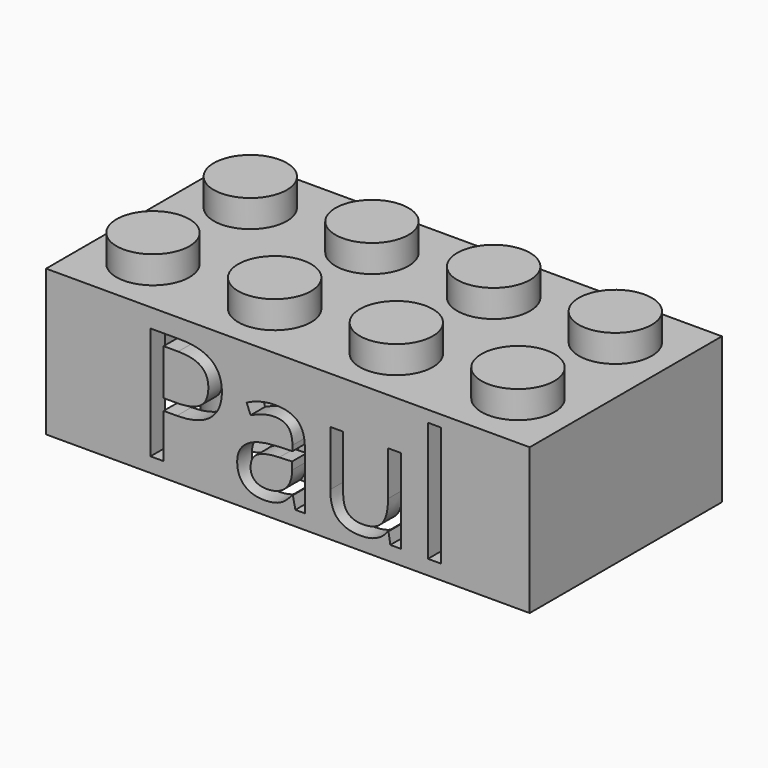
from build123d import *

# Parameters (mm, degrees)
F0_W          = 31.8
F0_H          = 15.8
F1_DEPTH      = 9.6
F2_W          = 29.4
F2_H          = 13.4
F3_DEPTH      = 8.4
F4_R          = 2.4
F5_DEPTH      = 1.8
F6_R          = 1.3
F7_DEPTH      = 1.2
F8_R          = 3.255
F8_R_2        = 2.4
F9_DEPTH      = 8.4
F10_W         = 0.6
F10_H         = 0.3
F11_DEPTH     = 8.4
F12_W         = 0.3
F12_H         = 0.6
F13_DEPTH     = 8.4
F14_W         = 0.6
F14_H         = 4
F15_DEPTH     = 6.4
F16_W         = 0.6
F16_H         = 4
F17_DEPTH     = 6.4
F18_TEXT_SIZE = 10.368521
F19_DEPTH     = 1.2


# Not quite as in the source:
# - Text() gives the source's letters only with a copy of the font that has no kerning and outlines rounded to 1/6400 em; it was checked with that copy


with BuildPart() as f1:
    # F0 (on Top) → F1 (new body)
    with BuildSketch(Plane.XY):
        Rectangle(F0_W, F0_H)
    extrude(amount=F1_DEPTH)

    # F2 (on face) → F3 (cut)
    with BuildSketch(Plane(origin=(0, 0, 0), x_dir=(1, 0, 0), z_dir=(0, 0, -1))):
        Rectangle(F2_W, F2_H)
    extrude(amount=-F3_DEPTH, mode=Mode.SUBTRACT)

    # F4 (on face) → F5 (join)
    with BuildSketch(Plane.XY.offset(9.6)):
        with Locations((-11.95, 3.95)):
            Circle(F4_R)
        with Locations((-11.95, -4.05)):
            Circle(F4_R)
        with Locations((-3.95, 3.95)):
            Circle(F4_R)
        with Locations((-3.95, -4.05)):
            Circle(F4_R)
        with Locations((4.05, 3.95)):
            Circle(F4_R)
        with Locations((4.05, -4.05)):
            Circle(F4_R)
        with Locations((12.05, 3.95)):
            Circle(F4_R)
        with Locations((12.05, -4.05)):
            Circle(F4_R)
    extrude(amount=F5_DEPTH)

    # F6 (on face) → F7 (cut)
    with BuildSketch(Plane(origin=(0, 0, 8.4), x_dir=(1, 0, 0), z_dir=(0, 0, -1))):
        with Locations((-11.95, 3.95)):
            Circle(F6_R)
        with Locations((-11.95, -4.05)):
            Circle(F6_R)
        with Locations((-3.95, 3.95)):
            Circle(F6_R)
        with Locations((-3.95, -4.05)):
            Circle(F6_R)
        with Locations((4.05, 3.95)):
            Circle(F6_R)
        with Locations((4.05, -4.05)):
            Circle(F6_R)
        with Locations((12.05, 3.95)):
            Circle(F6_R)
        with Locations((12.05, -4.05)):
            Circle(F6_R)
    extrude(amount=-F7_DEPTH, mode=Mode.SUBTRACT)

    # F8 (on face) → F9 (join, through all)
    with BuildSketch(Plane(origin=(0, 0, 8.4), x_dir=(1, 0, 0), z_dir=(0, 0, -1))):
        with Locations((-7.95, -0.05)):
            Circle(F8_R)
        with Locations((-7.95, -0.05)):
            Circle(F8_R_2, mode=Mode.SUBTRACT)
        with Locations((0.05, -0.05)):
            Circle(F8_R)
        with Locations((0.05, -0.05)):
            Circle(F8_R_2, mode=Mode.SUBTRACT)
        with Locations((8.05, -0.05)):
            Circle(F8_R)
        with Locations((8.05, -0.05)):
            Circle(F8_R_2, mode=Mode.SUBTRACT)
    extrude(amount=F9_DEPTH)

    # F10 (on face) → F11 (join, through all)
    with BuildSketch(Plane(origin=(0, 0, 0), x_dir=(1, 0, 0), z_dir=(0, 0, -1))):
        with Locations((-11.95, 6.55)):
            Rectangle(F10_W, F10_H)
        with Locations((-11.95, -6.55)):
            Rectangle(F10_W, F10_H)
        with Locations((-3.95, 6.55)):
            Rectangle(F10_W, F10_H)
        with Locations((-3.95, -6.55)):
            Rectangle(F10_W, F10_H)
        with Locations((4.05, 6.55)):
            Rectangle(F10_W, F10_H)
        with Locations((4.05, -6.55)):
            Rectangle(F10_W, F10_H)
        with Locations((12.05, 6.55)):
            Rectangle(F10_W, F10_H)
        with Locations((12.05, -6.55)):
            Rectangle(F10_W, F10_H)
    extrude(amount=-F11_DEPTH)

    # F12 (on face) → F13 (join, through all)
    with BuildSketch(Plane(origin=(0, 0, 0), x_dir=(1, 0, 0), z_dir=(0, 0, -1))):
        with Locations((-14.55, 4.05)):
            Rectangle(F12_W, F12_H)
        with Locations((-14.55, -3.95)):
            Rectangle(F12_W, F12_H)
        with Locations((14.55, 4.05)):
            Rectangle(F12_W, F12_H)
        with Locations((14.55, -3.95)):
            Rectangle(F12_W, F12_H)
    extrude(amount=-F13_DEPTH)

    # F14 (on face) → F15 (join)
    with BuildSketch(Plane(origin=(0, 0, 8.4), x_dir=(1, 0, 0), z_dir=(0, 0, -1))):
        with Locations((0, 4.876559)):
            Rectangle(F14_W, F14_H)
    extrude(amount=F15_DEPTH)

    # F16 (on face) → F17 (join)
    with BuildSketch(Plane(origin=(0, 0, 8.4), x_dir=(1, 0, 0), z_dir=(0, 0, -1))):
        with Locations((0, -5.091144)):
            Rectangle(F16_W, F16_H)
    extrude(amount=F17_DEPTH)

    # F18 (on face) → F19 (cut)
    with BuildSketch(Plane.XZ.offset(7.9)):
        with Locations((-10.051795, 0.966596)):
            Text('Paul', F18_TEXT_SIZE, font='Open Sans', text_align=(TextAlign.LEFT, TextAlign.BOTTOM))
    extrude(amount=-F19_DEPTH, mode=Mode.SUBTRACT)


solid = f1.part
